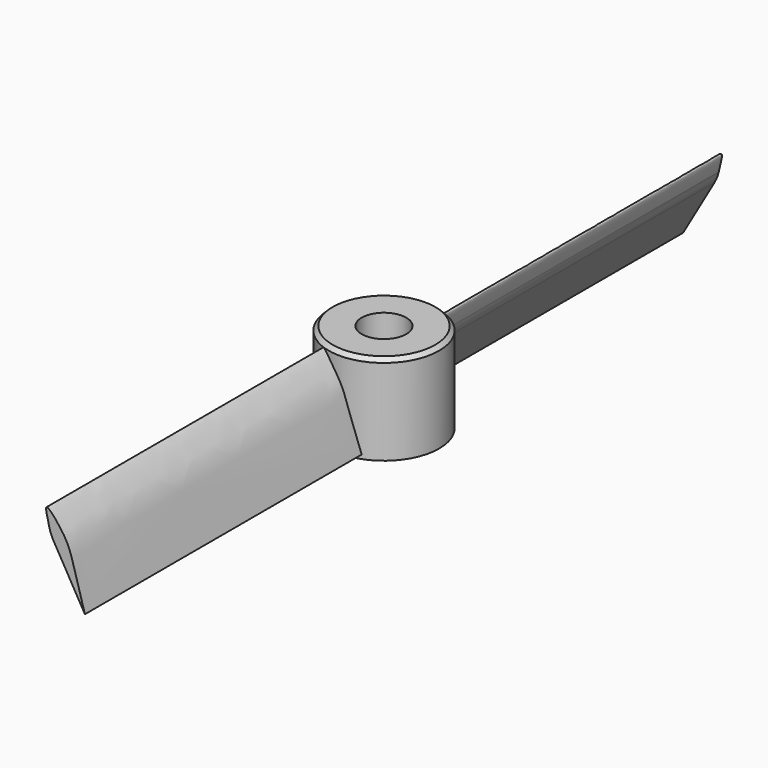
from build123d import *

# Parameters (mm, degrees)
F0_R     = 7.05
F0_R_2   = 2.85
F1_DEPTH = 11.5
F3_DEPTH = 50.8
F4_R     = 5
F6_DEPTH = 50.8
F7_R     = 5
F8_SIZE  = 0.5
F9_DEPTH = 25


# Not quite as in the source:
# - a feature names something its author has since deleted; it is built from what else it names


with BuildPart() as f1:
    # F0 (on Top) → F1 (new body)
    with BuildSketch(Plane.XY):
        Circle(F0_R)
        Circle(F0_R_2, mode=Mode.SUBTRACT)
        Circle(F0_R_2)
    extrude(amount=F1_DEPTH)

    # F2 (on Front) → F3 (join)
    with BuildSketch(Plane.XZ):
        with BuildLine():
            add(Edge.make_bspline(
                [(-1.9692358737, 8.16406228), (-2.2423085356, 9.5880753328), (-3.1767915601, 12.2160323736), (-0.2051875068, 8.7655282214), (0.7050474469, 6.7009656487), (1.5502972381, 3.5094202154), (2.1394422531, 1.5160002409), (2.4392272283, 0.5190588086)],
                knots=[0, 0, 0, 0, 0.1977876363, 0.3919769243, 0.5835513721, 0.7917756861, 1, 1, 1, 1], degree=3))
            Line((-1.9692358737, 8.16406228), (2.4392272283, 0.5190588086))
        make_face()
    extrude(amount=F3_DEPTH)

    # F4
    f4_edges = [f1.edges().sort_by_distance(p)[0] for p in [
        (-1.969236, -28.784694, 8.164062),
    ]]
    fillet(f4_edges, radius=F4_R)

    # F5 (on Front) → F6 (join)
    with BuildSketch(Plane.XZ):
        with BuildLine():
            Line((-2.4392190137, 0.5190687071), (1.9692440883, 8.1640721785))
            add(Edge.make_bspline(
                [(1.9692440883, 8.1640721785), (2.2423167503, 9.5880852313), (3.1767997747, 12.2160422721), (0.2051957214, 8.7655381198), (-0.7050392323, 6.7009755471), (-1.5502890235, 3.5094301139), (-2.1394340385, 1.5160101393), (-2.4392190137, 0.5190687071)],
                knots=[0, 0, 0, 0, 0.1977876363, 0.3919769243, 0.5835513721, 0.7917756861, 1, 1, 1, 1], degree=3))
        make_face()
    extrude(amount=-F6_DEPTH)

    # F7
    f7_edges = [f1.edges().sort_by_distance(p)[0] for p in [
        (1.969244, 28.784693, 8.164072),
    ]]
    fillet(f7_edges, radius=F7_R)

    # F8
    f8_edges = [f1.edges().sort_by_distance(p)[0] for p in [
        (-7.05, 0, 11.5),
    ]]
    chamfer(f8_edges, length=F8_SIZE)

    # F0 (on Top) → F9 (cut)
    with BuildSketch(Plane.XY):
        Circle(F0_R_2)
    extrude(amount=F9_DEPTH, mode=Mode.SUBTRACT)


solid = f1.part
